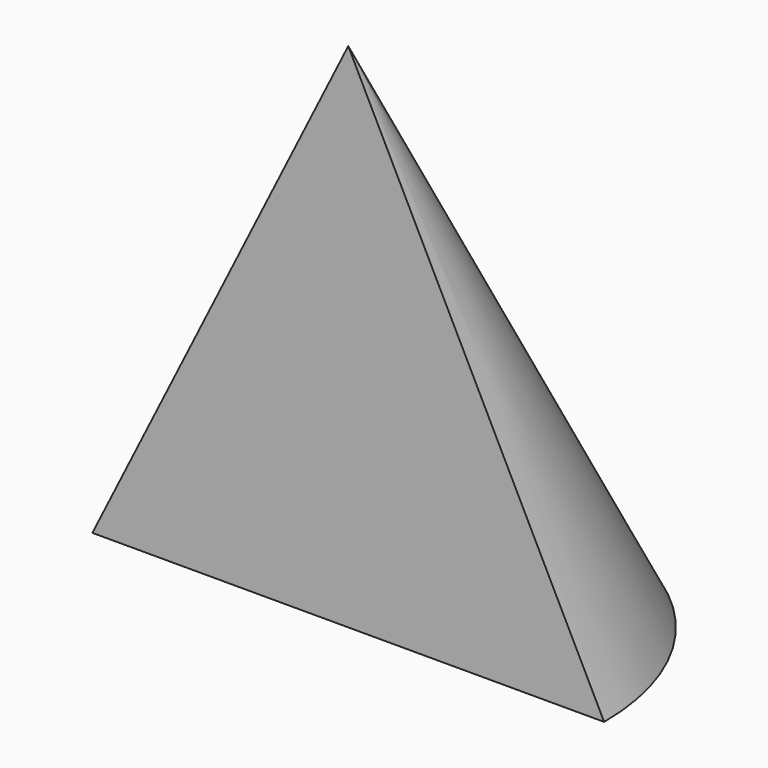
from build123d import *

# Parameters (mm, degrees)
F0_R     = 25.4
F1_DEPTH = 50.8
F2_SIZE2 = 50.79999
F2_SIZE  = 25.39999
F3_W     = 50.8
F3_H     = 25.4
F4_DEPTH = 101


# Not quite as in the source:
# - a fillet or chamfer is up to 0.001 mm smaller than in the source, because OpenCascade refuses the exact size
# - an extrude ends at something that could not be found from the text; its depth is read off the source's solid


with BuildPart() as f1:
    # F0 (on Top) → F1 (new body)
    with BuildSketch(Plane.XY):
        Circle(F0_R)
    extrude(amount=F1_DEPTH)

    # F2 (size 25.4 and 50.8 in the source; OpenCascade refuses exactly that, so slightly less here)
    f2_edges = [f1.edges().sort_by_distance(p)[0] for p in [
        (-25.4, 0, 50.8),
    ]]
    f2_side = f1.faces().sort_by_distance((0, 0, 50.8))[0]
    chamfer(f2_edges, length=F2_SIZE, length2=F2_SIZE2, reference=f2_side)

    # F3 (on face) → F4 (cut, through all)
    with BuildSketch(Plane(origin=(0, 0, 0), x_dir=(1, 0, 0), z_dir=(0, 0, -1))):
        with Locations((0, 12.7)):
            Rectangle(F3_W, F3_H)
    extrude(amount=-F4_DEPTH, mode=Mode.SUBTRACT)


solid = f1.part
